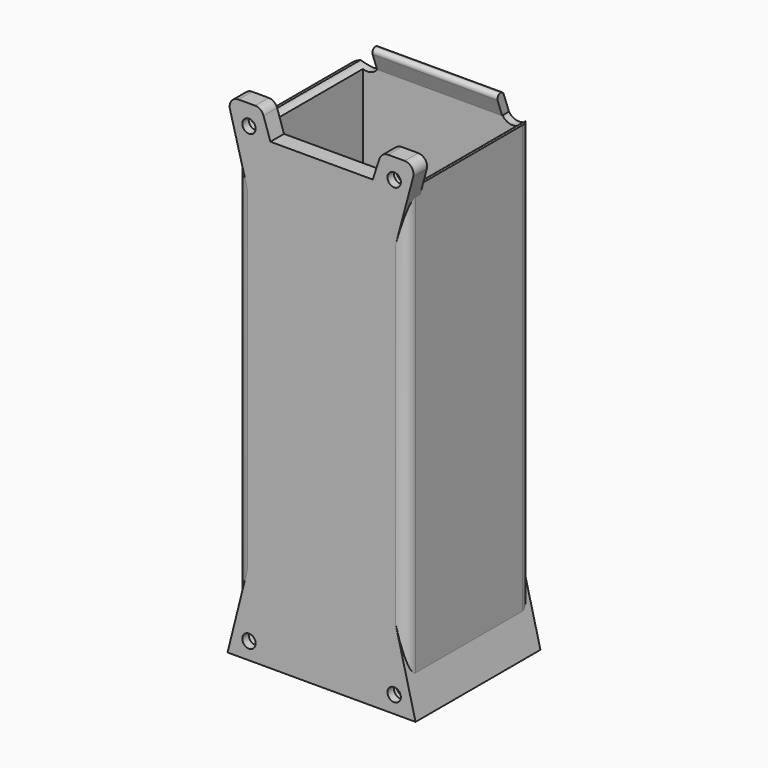
from build123d import *

# Parameters (mm, degrees)
F3_W           = 38.1
F3_H           = 32.95
F3_W_2         = 34.5
F3_H_2         = 29.35
F4_DEPTH       = 102
F6_W           = 5.6
F6_H           = 6
F7_DEPTH       = 1.8
F5_R           = 1.5
F9_DEPTH       = 2
F10_DEPTH      = 32.951
F10_DEPTH_BACK = 25
F11_W          = 38.1
F11_H          = 34.95
F12_DEPTH      = 1.8
F14_DEPTH      = 3.8
F15_R          = 2.7
F16_DEPTH      = 2
F16_DEPTH_BACK = 31.151
F17_DEPTH      = 31.15
F19_DEPTH      = 25
F20_R          = 2.5
F21_R          = 2
F24_DEPTH      = 28
F25_R          = 0.89999


# Not quite as in the source:
# - a fillet or chamfer is up to 0.001 mm smaller than in the source, because OpenCascade refuses the exact size


with BuildPart() as f4:
    # F3 (on Top) → F4 (new body)
    with BuildSketch(Plane.XY):
        Rectangle(F3_W, F3_H)
        Rectangle(F3_W_2, F3_H_2, mode=Mode.SUBTRACT)
    extrude(amount=F4_DEPTH)


with BuildPart() as f7:
    # F6 (on face) → F7 (new body)
    with BuildSketch(Plane.XZ.offset(16.475)):
        with Locations((-16.25, 105)):
            Rectangle(F6_W, F6_H)
    extrude(amount=-F7_DEPTH)


with BuildPart() as f7b:
    # F6 (on face) → F7, piece 2 (new body)
    with BuildSketch(Plane.XZ.offset(16.475)):
        with Locations((16.25, 105)):
            Rectangle(F6_W, F6_H)
    extrude(amount=-F7_DEPTH)


with BuildPart() as f4_1:
    add(f4.part)

    # F8: union F7, F7b
    add(f7.part)
    add(f7b.part)

    # F5 (on face) + F8_face (on face) → F9 (join)
    with BuildSketch(Plane.XZ.offset(16.475)):
        Polygon((16.25, 102), (-16.2500000167, 102), (-19.05, 102), (-19.05, 0), (19.05, 0), (19.05, 102), align=None)
        with Locations((-16.25, 2)):
            Circle(F5_R, mode=Mode.SUBTRACT)
        with Locations((16.25, 2)):
            Circle(F5_R, mode=Mode.SUBTRACT)
    with BuildSketch(Plane(origin=(0, -16.475, 51.9178934588), x_dir=(1, 0, 0), z_dir=(0, -1, 0))):
        Polygon((-19.05, 56.0821065412), (-19.05, -51.9178934588), (19.05, -51.9178934588), (19.05, 56.0821065412), (13.45, 56.0821065412), (13.45, 50.0821065412), (-13.45, 50.0821065412), (-13.45, 56.0821065412), align=None)
    extrude(amount=F9_DEPTH)

    # F5 (on face) → F10 (cut, two sides)
    with BuildSketch(Plane.XZ.offset(16.475)) as f10_sk:
        with Locations((-16.25, 2)):
            Circle(F5_R)
        with Locations((-16.25, 103.5)):
            Circle(F5_R)
        with Locations((16.25, 103.5)):
            Circle(F5_R)
        with Locations((16.25, 2)):
            Circle(F5_R)
    extrude(amount=-F10_DEPTH, mode=Mode.SUBTRACT)
    extrude(f10_sk.sketch, amount=F10_DEPTH_BACK, mode=Mode.SUBTRACT)

    # F11 (on face) → F12 (join)
    with BuildSketch(Plane(origin=(0, 0, 0), x_dir=(1, 0, 0), z_dir=(0, 0, -1))):
        with Locations((0, 1)):
            Rectangle(F11_W, F11_H)
    extrude(amount=F12_DEPTH)

    # F13 (on face) → F14 (join)
    with BuildSketch(Plane.XZ.offset(18.475)):
        Polygon((-19.05, 100), (-19.05, 108), (-21.1935935394, 108), align=None)
        Polygon((-21.05, -1.8), (-19.05, -1.8), (-19.05, 6.2), align=None)
        Polygon((21.05, -1.8), (19.05, 6.2), (19.05, -1.8), align=None)
        Polygon((21.1935935394, 108), (19.05, 108), (19.05, 100), align=None)
        Polygon((13.45, 102), (13.45, 108), (11.45, 102), align=None)
        Polygon((-13.45, 102), (-11.45, 102), (-13.45, 108), align=None)
    extrude(amount=-F14_DEPTH)

    # F15 (on face) → F16 (cut, two sides)
    with BuildSketch(Plane(origin=(0, -14.675, 0), x_dir=(-1, 0, 0), z_dir=(0, 1, 0))) as f16_sk:
        with Locations((-16.25, 103.5)):
            Circle(F15_R)
        with Locations((16.25, 103.5)):
            Circle(F15_R)
        with Locations((-16.25, 2)):
            Circle(F15_R)
        with Locations((16.25, 2)):
            Circle(F15_R)
    extrude(amount=-F16_DEPTH, mode=Mode.SUBTRACT)
    extrude(f16_sk.sketch, amount=F16_DEPTH_BACK, mode=Mode.SUBTRACT)

    # F17 (add, through all): faces of the model
    f17_faces = [f4_1.faces().sort_by_distance(p)[0] for p in [
        (-19.7166666667, -14.675, 0.8666666667),
        (19.7166666667, -14.675, 0.8666666667),
    ]]
    extrude(f17_faces, amount=F17_DEPTH)

    # F18 (on face) → F19 (cut)
    with BuildSketch(Plane(origin=(0, 0, -1.8), x_dir=(1, 0, 0), z_dir=(0, 0, -1))):
        with BuildLine():
            Line((10, 9.9949482828), (0, 9.9949482828))
            Line((0, 9.9949482828), (0, 0))
            Line((0, 0), (15, 0))
            Line((15, 0), (15, 4.9949482828))
            ThreePointArc((15, 4.9949482828), (13.5355339059, 8.5304821888), (10, 9.9949482828))
        make_face()
        with BuildLine():
            Line((0, 0), (0, 9.9949482828))
            Line((0, 9.9949482828), (-10, 9.9949482828))
            ThreePointArc((-10, 9.9949482828), (-13.5355339059, 8.5304821888), (-15, 4.9949482828))
            Line((-15, 4.9949482828), (-15, 0))
            Line((-15, 0), (0, 0))
        make_face()
        with BuildLine():
            Line((15, 0), (0, 0))
            Line((0, 0), (0, -9.9949482828))
            Line((0, -9.9949482828), (10, -9.9949482828))
            ThreePointArc((10, -9.9949482828), (13.5355339059, -8.5304821888), (15, -4.9949482828))
            Line((15, -4.9949482828), (15, 0))
        make_face()
        with BuildLine():
            Line((0, -9.9949482828), (0, 0))
            Line((0, 0), (-15, 0))
            Line((-15, 0), (-15, -4.9949482828))
            ThreePointArc((-15, -4.9949482828), (-13.5355339059, -8.5304821888), (-10, -9.9949482828))
            Line((-10, -9.9949482828), (0, -9.9949482828))
        make_face()
    extrude(amount=-F19_DEPTH, mode=Mode.SUBTRACT)

    # F20
    f20_edges = [f4_1.edges().sort_by_distance(p)[0] for p in [
        (-19.05, 16.475, 54.1),
        (19.05, 16.475, 54.1),
        (19.05, -18.475, 53.1),
        (-19.05, -18.475, 53.1),
    ]]
    fillet(f20_edges, radius=F20_R)

    # F21
    f21_edges = [f4_1.edges().sort_by_distance(p)[0] for p in [
        (-13.45, -16.575, 108),
        (-21.193594, -16.575, 108),
        (13.45, -16.575, 108),
        (21.193594, -16.575, 108),
    ]]
    fillet(f21_edges, radius=F21_R)

    # F23 (on face) → F24 (join)
    with BuildSketch(Plane.YZ.offset(14.0050055679)):
        Polygon((14.5708874184, 101.9686584017), (16.475, 102), (14.7648992834, 106.6984631039), (12.8493792929, 106.6984631039), align=None)
    extrude(amount=-F24_DEPTH)

    # F25 (radius 0.9 in the source; OpenCascade refuses exactly that, so slightly less here)
    f25_edges = [f4_1.edges().sort_by_distance(p)[0] for p in [
        (0.005006, 14.764899, 106.698463),
        (0.005006, 12.849379, 106.698463),
    ]]
    fillet(f25_edges, radius=F25_R)


solid = f4_1.part
